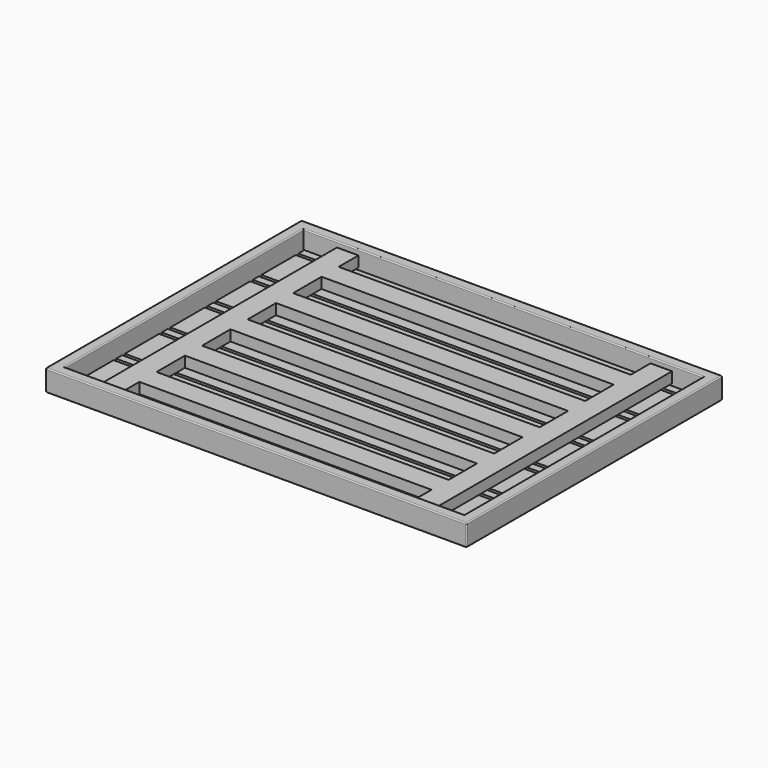
from build123d import *

# Parameters (mm, degrees)
F0_W     = 1960
F0_H     = 1490
F0_W_2   = 1860
F0_H_2   = 1390
F1_DEPTH = 100
F2_DEPTH = 25
F0_W_3   = 1830
F0_H_3   = 200
F0_H_4   = 35
F3_R     = 5
F4_R     = 5
F5_W     = 1360
F5_H     = 165
F6_DEPTH = 50


# Not quite as in the source:
# - a feature names something its author has since deleted; it is built from what else it names


with BuildPart() as f1:
    # F0 (on Top) → F1 (new body)
    with BuildSketch(Plane.XY):
        with Locations((980, 745)):
            Rectangle(F0_W, F0_H)
        with Locations((980, 745)):
            Rectangle(F0_W_2, F0_H_2, mode=Mode.SUBTRACT)
    extrude(amount=F1_DEPTH)

    # F0 (on Top) → F2 (join)
    with BuildSketch(Plane.XY):
        with Locations((980, 745)):
            Rectangle(F0_W, F0_H)
        with Locations((980, 745)):
            Rectangle(F0_W_2, F0_H_2, mode=Mode.SUBTRACT)
    extrude(amount=F2_DEPTH)

    # F3
    f3_edges = [f1.edges().sort_by_distance(p)[0] for p in [
        (980, 1440, 100),
        (50, 745, 100),
        (980, 50, 100),
        (1910, 745, 100),
    ]]
    fillet(f3_edges, radius=F3_R)

    # F4
    f4_edges = [f1.edges().sort_by_distance(p)[0] for p in [
        (980, 1490, 100),
        (0, 745, 100),
        (1960, 745, 100),
        (980, 0, 100),
        (1960, 0, 50),
        (0, 0, 50),
        (980, 0, 0),
        (0, 745, 0),
        (0, 1490, 50),
        (980, 1490, 0),
        (1960, 1490, 50),
        (1960, 745, 0),
        (50, 745, 0),
        (980, 1440, 0),
        (980, 50, 0),
        (1910, 745, 0),
    ]]
    fillet(f4_edges, radius=F4_R)


with BuildPart() as f2:
    # F0 (on Top) → F2, piece 2 (new body)
    with BuildSketch(Plane.XY):
        with Locations((980, 1275)):
            Rectangle(F0_W_3, F0_H_3)
    extrude(amount=F2_DEPTH)


with BuildPart() as f2b:
    # F0 (on Top) → F2, piece 3 (new body)
    with BuildSketch(Plane.XY):
        with Locations((980, 1010)):
            Rectangle(F0_W_3, F0_H_3)
    extrude(amount=F2_DEPTH)


with BuildPart() as f2c:
    # F0 (on Top) → F2, piece 4 (new body)
    with BuildSketch(Plane.XY):
        with Locations((980, 745)):
            Rectangle(F0_W_3, F0_H_3)
    extrude(amount=F2_DEPTH)


with BuildPart() as f2d:
    # F0 (on Top) → F2, piece 5 (new body)
    with BuildSketch(Plane.XY):
        with Locations((980, 480)):
            Rectangle(F0_W_3, F0_H_3)
    extrude(amount=F2_DEPTH)


with BuildPart() as f2e:
    # F0 (on Top) → F2, piece 6 (new body)
    with BuildSketch(Plane.XY):
        with Locations((980, 215)):
            Rectangle(F0_W_3, F0_H_3)
    extrude(amount=F2_DEPTH)


with BuildPart() as f2f:
    # F0 (on Top) → F2, piece 7 (new body)
    with BuildSketch(Plane.XY):
        with Locations((980, 82.5)):
            Rectangle(F0_W_3, F0_H_4)
    extrude(amount=F2_DEPTH)


with BuildPart() as f2g:
    # F0 (on Top) → F2, piece 8 (new body)
    with BuildSketch(Plane.XY):
        with Locations((980, 347.5)):
            Rectangle(F0_W_3, F0_H_4)
    extrude(amount=F2_DEPTH)


with BuildPart() as f2h:
    # F0 (on Top) → F2, piece 9 (new body)
    with BuildSketch(Plane.XY):
        with Locations((980, 612.5)):
            Rectangle(F0_W_3, F0_H_4)
    extrude(amount=F2_DEPTH)


with BuildPart() as f2i:
    # F0 (on Top) → F2, piece 10 (new body)
    with BuildSketch(Plane.XY):
        with Locations((980, 877.5)):
            Rectangle(F0_W_3, F0_H_4)
    extrude(amount=F2_DEPTH)


with BuildPart() as f2j:
    # F0 (on Top) → F2, piece 11 (new body)
    with BuildSketch(Plane.XY):
        with Locations((980, 1142.5)):
            Rectangle(F0_W_3, F0_H_4)
    extrude(amount=F2_DEPTH)


with BuildPart() as f2k:
    # F0 (on Top) → F2, piece 12 (new body)
    with BuildSketch(Plane.XY):
        with Locations((980, 1407.5)):
            Rectangle(F0_W_3, F0_H_4)
    extrude(amount=F2_DEPTH)


with BuildPart() as f6:
    # F5 (on face) → F6 (new body)
    with BuildSketch(Plane.XY.offset(25)):
        Polygon((205, 1440), (205, 50), (305, 50), (305, 165), (1665, 165), (1665, 50), (1765, 50), (1765, 1440), (1665, 1440), (1665, 1325), (305, 1325), (305, 1440), align=None)
        with Locations((985, 347.5)):
            Rectangle(F5_W, F5_H, mode=Mode.SUBTRACT)
        with Locations((985, 612.5)):
            Rectangle(F5_W, F5_H, mode=Mode.SUBTRACT)
        with Locations((985, 877.5)):
            Rectangle(F5_W, F5_H, mode=Mode.SUBTRACT)
        with Locations((985, 1142.5)):
            Rectangle(F5_W, F5_H, mode=Mode.SUBTRACT)
    extrude(amount=F6_DEPTH)


solid = Compound([f1.part, f2.part, f2b.part, f2c.part, f2d.part, f2e.part, f2f.part, f2g.part, f2h.part, f2i.part, f2j.part, f2k.part, f6.part])
